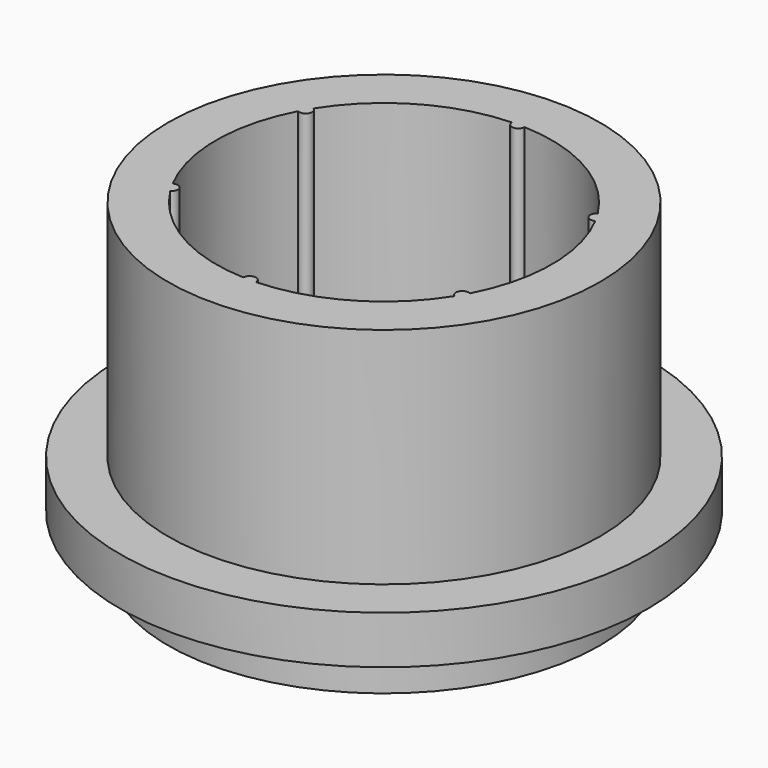
from build123d import *

# Parameters (mm, degrees)
F3_DEPTH        = 20
F3_COPIES_COUNT = 6


# Not quite as in the source:
# - a pattern or mirror of a feature is missing from the dataset's text; its kind, count and spacing are read off the source's solid


with BuildPart() as f1:
    # F0 (on Front) → F1 (revolve)
    with BuildSketch(Plane.XZ):
        Polygon((-13.5, -3), (-10.5, -3), (-10.5, 17), (-13.5, 17), (-13.5, 3), (-16.5, 3), (-16.5, 0), (-13.5, 0), align=None)
    revolve(axis=Axis((0, 0, 29.5368466722), (0, 0, 1)))

    # F2 (on face) → F3 (join, through all)
    with BuildSketch(Plane.XY.offset(17)):
        with BuildLine():
            ThreePointArc((0.3999274311, 10.4923809524), (0, 10.5), (-0.3999274311, 10.4923809524))
            ThreePointArc((-0.3999274311, 10.4923809524), (0, 10.1), (0.3999274311, 10.4923809524))
        make_face()
    f3 = extrude(amount=-F3_DEPTH)

    # F3_copies: F3 ×6 about axis
    f3_copies_axis = Axis((0, 0, 0), (0, 0, 1))
    for i in range(1, F3_COPIES_COUNT):
        add(f3.rotate(f3_copies_axis, i * 360 / F3_COPIES_COUNT))


solid = f1.part
